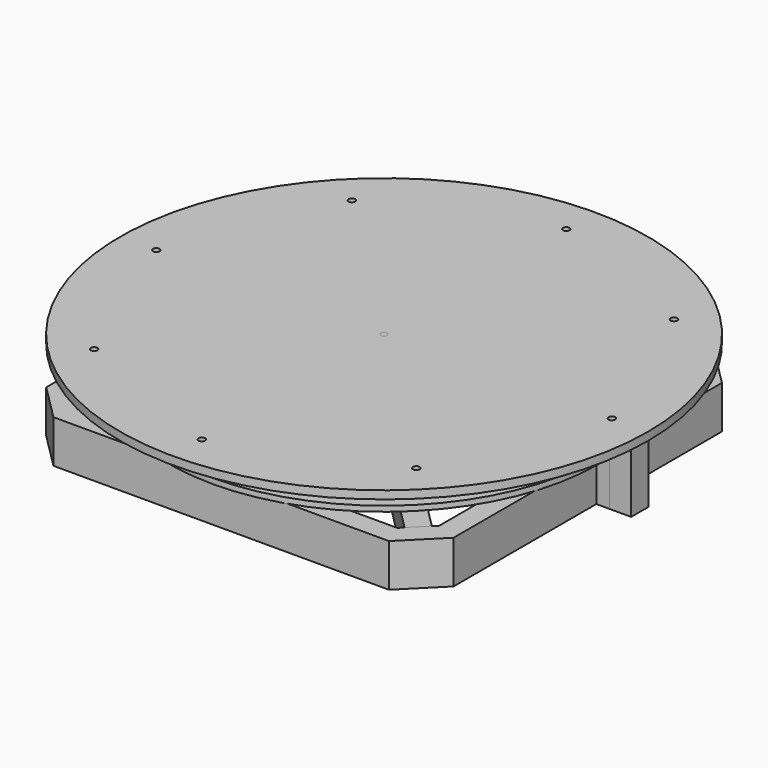
from build123d import *

# Parameters (mm, degrees)
F0_R      = 492.5
F0_R_2    = 6.25
F0_R_3    = 6
F1_DEPTH  = 15
F3_DEPTH  = 55
F4_R      = 5.1
F5_DEPTH  = 143.014158117
F6_COUNT  = 5
F10_START = 3
F9_R      = 23.5
F9_R_2    = 6
F10_DEPTH = 14
F11_SIZE  = 1
F12_COUNT = 5
F15_DEPTH = 10
F19_DEPTH = 80
F20_DEPTH = 60
F22_START = 10
F21_W     = 40
F21_H     = 40
F21_R     = 10
F22_DEPTH = 12
F23_START = 22
F23_DEPTH = 126.5
F24_W     = 40
F24_H     = 80
F25_DEPTH = 25
F26_COUNT = 2
F31_COUNT = 5


# Not quite as in the source:
# - a feature names something its author has since deleted; it is built from what else it names


with BuildPart() as f1:
    # F0 (on Top) → F1 (new body)
    with BuildSketch(Plane.XY):
        Circle(F0_R)
        with Locations((-300.5203820043, -300.5203820043)):
            Circle(F0_R_2, mode=Mode.SUBTRACT)
        with Locations((0, -425)):
            Circle(F0_R_2, mode=Mode.SUBTRACT)
        with Locations((300.5203820043, -300.5203820043)):
            Circle(F0_R_2, mode=Mode.SUBTRACT)
        with Locations((-425, 0)):
            Circle(F0_R_2, mode=Mode.SUBTRACT)
        with Locations((-300.5203820043, 300.5203820043)):
            Circle(F0_R_2, mode=Mode.SUBTRACT)
        Circle(F0_R_3, mode=Mode.SUBTRACT)
        with Locations((425, 0)):
            Circle(F0_R_2, mode=Mode.SUBTRACT)
        with Locations((0, 425)):
            Circle(F0_R_2, mode=Mode.SUBTRACT)
        with Locations((300.5203820043, 300.5203820043)):
            Circle(F0_R_2, mode=Mode.SUBTRACT)
    extrude(amount=F1_DEPTH)


with BuildPart() as f3:
    # F2 (on face) → F3 (new body)
    with BuildSketch(Plane(origin=(0, 0, 0), x_dir=(1, 0, 0), z_dir=(0, 0, -1))):
        Polygon((20, 379.486841883), (20, 389.486841883), (0, 389.486841883), (-20, 389.486841883), (-20, 379.486841883), (0, 379.486841883), align=None)
    extrude(amount=F3_DEPTH)


with BuildPart() as f3b:
    # F2 (on face) → F3, piece 2 (new body)
    with BuildSketch(Plane(origin=(0, 0, 0), x_dir=(1, 0, 0), z_dir=(0, 0, -1))):
        Polygon((-20, 349.486841883), (0, 349.486841883), (20, 349.486841883), (20, 359.486841883), (0, 359.486841883), (-20, 359.486841883), align=None)
    extrude(amount=F3_DEPTH)


with BuildPart() as f5_tool:
    # F4 (on face) → F5 (new body, through all)
    with BuildSketch(Plane(origin=(0, -349.486841883, 0), x_dir=(-1, 0, 0), z_dir=(0, 1, 0))):
        with Locations((0, -35)):
            Circle(F4_R)
        Polygon((20, -55), (20, -47.4944465005), (7, -55), align=None)
        Polygon((-20, -55), (-7, -55), (-20, -47.4944465005), align=None)
    extrude(amount=-F5_DEPTH)


with BuildPart() as f3_1:
    add(f3.part)

    # F5: cut by f5_tool
    add(f5_tool.part, mode=Mode.SUBTRACT)


with BuildPart() as f3b_1:
    add(f3b.part)

    # F5: cut by f5_tool
    add(f5_tool.part, mode=Mode.SUBTRACT)


with BuildPart() as f6_1:
    # F6: instance of F3b
    add(f3b_1.part.rotate(Axis((0, 0, 0), (0, 0, 1)), 1 * 360 / F6_COUNT))


with BuildPart() as f6_2:
    # F6: instance of F3b
    add(f3b_1.part.rotate(Axis((0, 0, 0), (0, 0, 1)), 2 * 360 / F6_COUNT))


with BuildPart() as f6_3:
    # F6: instance of F3b
    add(f3b_1.part.rotate(Axis((0, 0, 0), (0, 0, 1)), 3 * 360 / F6_COUNT))


with BuildPart() as f6_4:
    # F6: instance of F3b
    add(f3b_1.part.rotate(Axis((0, 0, 0), (0, 0, 1)), 4 * 360 / F6_COUNT))


with BuildPart() as f6_5:
    # F6: instance of F3
    add(f3_1.part.rotate(Axis((0, 0, 0), (0, 0, 1)), 1 * 360 / F6_COUNT))


with BuildPart() as f6_6:
    # F6: instance of F3
    add(f3_1.part.rotate(Axis((0, 0, 0), (0, 0, 1)), 2 * 360 / F6_COUNT))


with BuildPart() as f6_7:
    # F6: instance of F3
    add(f3_1.part.rotate(Axis((0, 0, 0), (0, 0, 1)), 3 * 360 / F6_COUNT))


with BuildPart() as f6_8:
    # F6: instance of F3
    add(f3_1.part.rotate(Axis((0, 0, 0), (0, 0, 1)), 4 * 360 / F6_COUNT))


with BuildPart() as f8:
    # F7 (on Front) → F8 (revolve)
    with BuildSketch(Plane.XZ):
        Polygon((6, 15), (0, 15), (0, -100), (16, -100), (20, -93.0717967697), (20, 0), (6, 0), align=None)
    revolve(axis=Axis((0, 0, -42.5), (0, 0, -1)))


with BuildPart() as f10:
    # F9 (on face) → F10 (new body)
    with BuildSketch(Plane.XZ.offset(359.486841883).offset(F10_START)):
        with Locations((0, -35)):
            Circle(F9_R)
        with Locations((0, -35)):
            Circle(F9_R_2, mode=Mode.SUBTRACT)
    extrude(amount=F10_DEPTH)

    # F11
    f11_edges = [f10.edges().sort_by_distance(p)[0] for p in [
        (-23.5, -376.486842, -35),
        (-23.5, -362.486842, -35),
    ]]
    chamfer(f11_edges, length=F11_SIZE)


with BuildPart() as f12_1:
    # F12: instance of F10
    add(f10.part.rotate(Axis((0, 0, -93.0717967697), (0, 0, 1)), 1 * 360 / F12_COUNT))


with BuildPart() as f12_2:
    # F12: instance of F10
    add(f10.part.rotate(Axis((0, 0, -93.0717967697), (0, 0, 1)), 2 * 360 / F12_COUNT))


with BuildPart() as f12_3:
    # F12: instance of F10
    add(f10.part.rotate(Axis((0, 0, -93.0717967697), (0, 0, 1)), 3 * 360 / F12_COUNT))


with BuildPart() as f12_4:
    # F12: instance of F10
    add(f10.part.rotate(Axis((0, 0, -93.0717967697), (0, 0, 1)), 4 * 360 / F12_COUNT))


with BuildPart() as f15:
    # F14 (on offset) → F15 (new body)
    with BuildSketch(Plane(origin=(0, 0, -58.5), x_dir=(1, 0, 0), z_dir=(0, 0, -1))):
        with BuildLine():
            ThreePointArc((-399.9999875, -0.1), (0, -400), (399.9999875, -0.1))
            Line((399.9999875, -0.1), (349.9999857143, -0.1))
            ThreePointArc((349.9999857143, -0.1), (0, -350), (-349.9999857143, -0.1))
            Line((-349.9999857143, -0.1), (-399.9999875, -0.1))
        make_face()
    extrude(amount=F15_DEPTH)


with BuildPart() as f15b:
    # F14 (on offset) → F15, piece 2 (new body)
    with BuildSketch(Plane(origin=(0, 0, -58.5), x_dir=(1, 0, 0), z_dir=(0, 0, -1))):
        with BuildLine():
            Line((349.9999857143, 0.1), (399.9999875, 0.1))
            ThreePointArc((399.9999875, 0.1), (0, 400), (-399.9999875, 0.1))
            Line((-399.9999875, 0.1), (-349.9999857143, 0.1))
            ThreePointArc((-349.9999857143, 0.1), (0, 350), (349.9999857143, 0.1))
        make_face()
    extrude(amount=F15_DEPTH)


with BuildPart() as f17:
    # F16 (on Front) → F17 (revolve)
    with BuildSketch(Plane.XZ):
        Polygon((24.1, -40), (20.1, -46.9282032303), (20.1, -128.5), (30, -128.5), (30, -40), align=None)
    revolve(axis=Axis((0, 0, -54.5029782762), (0, 0, -1)))


with BuildPart() as f19:
    # F18 (on face) → F19 (new body)
    with BuildSketch(Plane(origin=(0, 0, -68.5), x_dir=(1, 0, 0), z_dir=(0, 0, -1))):
        with BuildLine():
            Line((-349.9999857143, 0.1), (-380, 0.1))
            Line((-380, 0.1), (-380, -312.9646455009))
            Line((-380, -312.9646455009), (-312.9646456247, -380))
            Line((-312.9646456247, -380), (312.9646455009, -380))
            Line((312.9646455009, -380), (380, -312.9646456247))
            Line((380, -312.9646456247), (380, 0.1))
            Line((380, 0.1), (349.9999857143, 0.1))
            ThreePointArc((349.9999857143, 0.1), (347.4850273889, 41.8826424728), (340, 83.0662386292))
            Line((340, 83.0662386292), (340, -296.3961031082))
            Line((340, -296.3961031082), (332.3401868769, -304.0559162171))
            Line((332.3401868769, -304.0559162171), (304.0559156033, -332.3401874385))
            Line((304.0559156033, -332.3401874385), (296.3961030276, -340))
            Line((296.3961030276, -340), (-296.3961031082, -340))
            Line((-296.3961031082, -340), (-304.0559162171, -332.3401868769))
            Line((-304.0559162171, -332.3401868769), (-332.3401874385, -304.0559156033))
            Line((-332.3401874385, -304.0559156033), (-340, -296.3961030276))
            Line((-340, -296.3961030276), (-340, 83.0662386292))
            ThreePointArc((-340, 83.0662386292), (-347.4850273889, 41.8826424728), (-349.9999857143, 0.1))
        make_face()
        with BuildLine():
            Line((124.899959968, 380), (-124.899959968, 380))
            ThreePointArc((-124.899959968, 380), (-168.9941635669, 362.5478901888), (-210.7130750571, 340))
            Line((-210.7130750571, 340), (-83.0662386292, 340))
            ThreePointArc((-83.0662386292, 340), (0, 350), (83.0662386292, 340))
            Line((83.0662386292, 340), (210.7130750571, 340))
            ThreePointArc((210.7130750571, 340), (168.9941635669, 362.5478901888), (124.899959968, 380))
        make_face()
        with BuildLine():
            Line((312.9646456247, 380), (124.899959968, 380))
            ThreePointArc((124.899959968, 380), (168.9941635669, 362.5478901888), (210.7130750571, 340))
            Line((210.7130750571, 340), (296.3961031082, 340))
            Line((296.3961031082, 340), (304.0559162171, 332.3401868769))
            Line((304.0559162171, 332.3401868769), (332.3401874385, 304.0559156033))
            Line((332.3401874385, 304.0559156033), (340, 296.3961030276))
            Line((340, 296.3961030276), (340, 210.7130750571))
            ThreePointArc((340, 210.7130750571), (362.5478901888, 168.9941635669), (380, 124.899959968))
            Line((380, 124.899959968), (380, 312.9646455009))
            Line((380, 312.9646455009), (312.9646456247, 380))
        make_face()
        with BuildLine():
            ThreePointArc((-340, 210.7130750571), (-362.5478901888, 168.9941635669), (-380, 124.899959968))
            Line((-380, 124.899959968), (-380, 0.1))
            Line((-380, 0.1), (-349.9999857143, 0.1))
            ThreePointArc((-349.9999857143, 0.1), (-347.4850273889, 41.8826424728), (-340, 83.0662386292))
            Line((-340, 83.0662386292), (-340, 210.7130750571))
        make_face()
        with BuildLine():
            Line((-124.899959968, 380), (-312.9646455009, 380))
            Line((-312.9646455009, 380), (-380, 312.9646456247))
            Line((-380, 312.9646456247), (-380, 124.899959968))
            ThreePointArc((-380, 124.899959968), (-362.5478901888, 168.9941635669), (-340, 210.7130750571))
            Line((-340, 210.7130750571), (-340, 296.3961031082))
            Line((-340, 296.3961031082), (-332.3401868769, 304.0559162171))
            Line((-332.3401868769, 304.0559162171), (-304.0559156033, 332.3401874385))
            Line((-304.0559156033, 332.3401874385), (-296.3961030276, 340))
            Line((-296.3961030276, 340), (-210.7130750571, 340))
            ThreePointArc((-210.7130750571, 340), (-168.9941635669, 362.5478901888), (-124.899959968, 380))
        make_face()
        with BuildLine():
            Line((380, 0.1), (380, 124.899959968))
            ThreePointArc((380, 124.899959968), (362.5478901888, 168.9941635669), (340, 210.7130750571))
            Line((340, 210.7130750571), (340, 83.0662386292))
            ThreePointArc((340, 83.0662386292), (347.4850273889, 41.8826424728), (349.9999857143, 0.1))
            Line((349.9999857143, 0.1), (380, 0.1))
        make_face()
        with BuildLine():
            ThreePointArc((83.0662386292, 340), (0, 350), (-83.0662386292, 340))
            Line((-83.0662386292, 340), (83.0662386292, 340))
        make_face()
    extrude(amount=F19_DEPTH)


with BuildPart() as f20:
    # F18 (on face) → F20 (new body)
    with BuildSketch(Plane(origin=(0, 0, -68.5), x_dir=(1, 0, 0), z_dir=(0, 0, -1))):
        with BuildLine():
            Line((-232.9408461471, 261.225117851), (-268.3468019388, 296.6310737081))
            ThreePointArc((-268.3468019388, 296.6310737081), (-282.8427122134, 282.8427127358), (-296.6310732124, 268.3468024867))
            Line((-296.6310732124, 268.3468024867), (-261.2251174207, 232.9408466296))
            ThreePointArc((-261.2251174207, 232.9408466296), (-247.4873731867, 247.4873736439), (-232.9408461471, 261.225117851))
        make_face()
        with BuildLine():
            ThreePointArc((-296.6310732124, 268.3468024867), (-282.8427122134, 282.8427127358), (-268.3468019388, 296.6310737081))
            Line((-268.3468019388, 296.6310737081), (-304.0559156033, 332.3401874385))
            Line((-304.0559156033, 332.3401874385), (-332.3401868769, 304.0559162171))
            Line((-332.3401868769, 304.0559162171), (-296.6310732124, 268.3468024867))
        make_face()
        with BuildLine():
            Line((-3.33642264, 31.6206939198), (-232.9408461471, 261.225117851))
            ThreePointArc((-232.9408461471, 261.225117851), (-247.4873731867, 247.4873736439), (-261.2251174207, 232.9408466296))
            Line((-261.2251174207, 232.9408466296), (-31.6206939136, 3.3364226984))
            Line((-31.6206939136, 3.3364226984), (-29.4993735681, 5.45774304))
            ThreePointArc((-29.4993735681, 5.45774304), (-21.213203416, 21.2132034552), (-5.4577429855, 29.4993735782))
            Line((-5.4577429855, 29.4993735782), (-3.33642264, 31.6206939198))
        make_face()
    extrude(amount=F20_DEPTH)


with BuildPart() as f20b:
    # F18 (on face) → F20, piece 2 (new body)
    with BuildSketch(Plane(origin=(0, 0, -68.5), x_dir=(1, 0, 0), z_dir=(0, 0, -1))):
        with BuildLine():
            ThreePointArc((296.6310737081, 268.3468019388), (282.8427127358, 282.8427122134), (268.3468024867, 296.6310732124))
            Line((268.3468024867, 296.6310732124), (232.9408466296, 261.2251174207))
            ThreePointArc((232.9408466296, 261.2251174207), (247.4873736439, 247.4873731867), (261.225117851, 232.9408461471))
            Line((261.225117851, 232.9408461471), (296.6310737081, 268.3468019388))
        make_face()
        with BuildLine():
            Line((304.0559162171, 332.3401868769), (268.3468024867, 296.6310732124))
            ThreePointArc((268.3468024867, 296.6310732124), (282.8427127358, 282.8427122134), (296.6310737081, 268.3468019388))
            Line((296.6310737081, 268.3468019388), (332.3401874385, 304.0559156033))
            Line((332.3401874385, 304.0559156033), (304.0559162171, 332.3401868769))
        make_face()
        with BuildLine():
            ThreePointArc((261.225117851, 232.9408461471), (247.4873736439, 247.4873731867), (232.9408466296, 261.2251174207))
            Line((232.9408466296, 261.2251174207), (3.3364226984, 31.6206939136))
            Line((3.3364226984, 31.6206939136), (5.45774304, 29.4993735681))
            ThreePointArc((5.45774304, 29.4993735681), (21.2132034552, 21.213203416), (29.4993735782, 5.4577429855))
            Line((29.4993735782, 5.4577429855), (31.6206939198, 3.33642264))
            Line((31.6206939198, 3.33642264), (261.225117851, 232.9408461471))
        make_face()
    extrude(amount=F20_DEPTH)


with BuildPart() as f20c:
    # F18 (on face) → F20, piece 3 (new body)
    with BuildSketch(Plane(origin=(0, 0, -68.5), x_dir=(1, 0, 0), z_dir=(0, 0, -1))):
        with BuildLine():
            Line((304.0559156033, -332.3401874385), (332.3401868769, -304.0559162171))
            Line((332.3401868769, -304.0559162171), (31.6206939136, -3.3364226984))
            Line((31.6206939136, -3.3364226984), (29.4993735681, -5.45774304))
            ThreePointArc((29.4993735681, -5.45774304), (21.213203416, -21.2132034552), (5.4577429855, -29.4993735782))
            Line((5.4577429855, -29.4993735782), (3.33642264, -31.6206939198))
            Line((3.33642264, -31.6206939198), (304.0559156033, -332.3401874385))
        make_face()
    extrude(amount=F20_DEPTH)


with BuildPart() as f20d:
    # F18 (on face) → F20, piece 4 (new body)
    with BuildSketch(Plane(origin=(0, 0, -68.5), x_dir=(1, 0, 0), z_dir=(0, 0, -1))):
        with BuildLine():
            Line((-31.6206939198, -3.33642264), (-332.3401874385, -304.0559156033))
            Line((-332.3401874385, -304.0559156033), (-304.0559162171, -332.3401868769))
            Line((-304.0559162171, -332.3401868769), (-3.3364226984, -31.6206939136))
            Line((-3.3364226984, -31.6206939136), (-5.45774304, -29.4993735681))
            ThreePointArc((-5.45774304, -29.4993735681), (-21.2132034552, -21.213203416), (-29.4993735782, -5.4577429855))
            Line((-29.4993735782, -5.4577429855), (-31.6206939198, -3.33642264))
        make_face()
    extrude(amount=F20_DEPTH)


with BuildPart() as f22:
    # F21 (on face) → F22 (new body)
    with BuildSketch(Plane(origin=(0, 0, 0), x_dir=(1, 0, 0), z_dir=(0, 0, -1)).offset(F22_START)):
        with Locations((425, -40)):
            Rectangle(F21_W, F21_H)
        with Locations((425, 0)):
            Rectangle(F21_W, F21_H)
        with Locations((425, 0)):
            Circle(F21_R, mode=Mode.SUBTRACT)
    extrude(amount=F22_DEPTH)


with BuildPart() as f23:
    # F21 (on face) → F23 (new body)
    with BuildSketch(Plane(origin=(0, 0, 0), x_dir=(1, 0, 0), z_dir=(0, 0, -1)).offset(F23_START)):
        with Locations((425, -40)):
            Rectangle(F21_W, F21_H)
    extrude(amount=F23_DEPTH)


with BuildPart() as f25:
    # F24 (on face) → F25 (new body)
    with BuildSketch(Plane(origin=(405, 0, 0), x_dir=(0, -1, 0), z_dir=(-1, 0, 0))):
        with Locations((-40, -108.5)):
            Rectangle(F24_W, F24_H)
    extrude(amount=F25_DEPTH)


with BuildPart() as f26_1:
    # F26: instance of F23
    add(f23.part.rotate(Axis((0, 0, -93.0717967697), (0, 0, 1)), 1 * 360 / F26_COUNT))


with BuildPart() as f26_2:
    # F26: instance of F25
    add(f25.part.rotate(Axis((0, 0, -93.0717967697), (0, 0, 1)), 1 * 360 / F26_COUNT))


with BuildPart() as f26_3:
    # F26: instance of F22
    add(f22.part.rotate(Axis((0, 0, -93.0717967697), (0, 0, 1)), 1 * 360 / F26_COUNT))


with BuildPart() as f29:
    # F28 (on offset) → F29 (revolve)
    with BuildSketch(Plane(origin=(0, 0, -35), x_dir=(1, 0, 0), z_dir=(0, 0, -1))):
        Polygon((-5, 371.486841883), (-5, 379.486841883), (-11, 379.486841883), (-11, 376.486841883), (-8.45, 376.486841883), (-8.45, 371.486841883), align=None)
    revolve(axis=Axis((0, -379.0543241254, -35), (0, -1, 0)))


with BuildPart() as f29b:
    # F28 (on offset) → F29, piece 2 (revolve)
    with BuildSketch(Plane(origin=(0, 0, -35), x_dir=(1, 0, 0), z_dir=(0, 0, -1))):
        Polygon((-5, 367.486841883), (-8.45, 367.486841883), (-8.45, 362.486841883), (-11, 362.486841883), (-11, 359.486841883), (-5, 359.486841883), align=None)
    revolve(axis=Axis((0, -379.0543241254, -35), (0, -1, 0)))


with BuildPart() as f30:
    # F28 (on offset) → F30 (revolve)
    with BuildSketch(Plane(origin=(0, 0, -35), x_dir=(1, 0, 0), z_dir=(0, 0, -1))):
        Polygon((-5, 371.486841883), (-5, 379.486841883), (-11, 379.486841883), (-11, 376.486841883), (-8.45, 376.486841883), (-8.45, 371.486841883), align=None)
    revolve(axis=Axis((0, -379.0543241254, -35), (0, -1, 0)))


with BuildPart() as f31_1:
    # F31: instance of F29
    add(f29.part.rotate(Axis((0, 0, -100), (0, 0, -1)), 1 * 360 / F31_COUNT))


with BuildPart() as f31_2:
    # F31: instance of F29
    add(f29.part.rotate(Axis((0, 0, -100), (0, 0, -1)), 2 * 360 / F31_COUNT))


with BuildPart() as f31_3:
    # F31: instance of F29
    add(f29.part.rotate(Axis((0, 0, -100), (0, 0, -1)), 3 * 360 / F31_COUNT))


with BuildPart() as f31_4:
    # F31: instance of F29
    add(f29.part.rotate(Axis((0, 0, -100), (0, 0, -1)), 4 * 360 / F31_COUNT))


with BuildPart() as f31_5:
    # F31: instance of F29b
    add(f29b.part.rotate(Axis((0, 0, -100), (0, 0, -1)), 1 * 360 / F31_COUNT))


with BuildPart() as f31_6:
    # F31: instance of F29b
    add(f29b.part.rotate(Axis((0, 0, -100), (0, 0, -1)), 2 * 360 / F31_COUNT))


with BuildPart() as f31_7:
    # F31: instance of F29b
    add(f29b.part.rotate(Axis((0, 0, -100), (0, 0, -1)), 3 * 360 / F31_COUNT))


with BuildPart() as f31_8:
    # F31: instance of F29b
    add(f29b.part.rotate(Axis((0, 0, -100), (0, 0, -1)), 4 * 360 / F31_COUNT))


solid = Compound([f1.part, f3_1.part, f3b_1.part, f6_1.part, f6_2.part, f6_3.part, f6_4.part, f6_5.part, f6_6.part, f6_7.part, f6_8.part, f8.part, f10.part, f12_1.part, f12_2.part, f12_3.part, f12_4.part, f15.part, f15b.part, f17.part, f19.part, f20.part, f20b.part, f20c.part, f20d.part, f22.part, f23.part, f25.part, f26_1.part, f26_2.part, f26_3.part, f29.part, f29b.part, f30.part, f31_1.part, f31_2.part, f31_3.part, f31_4.part, f31_5.part, f31_6.part, f31_7.part, f31_8.part])
